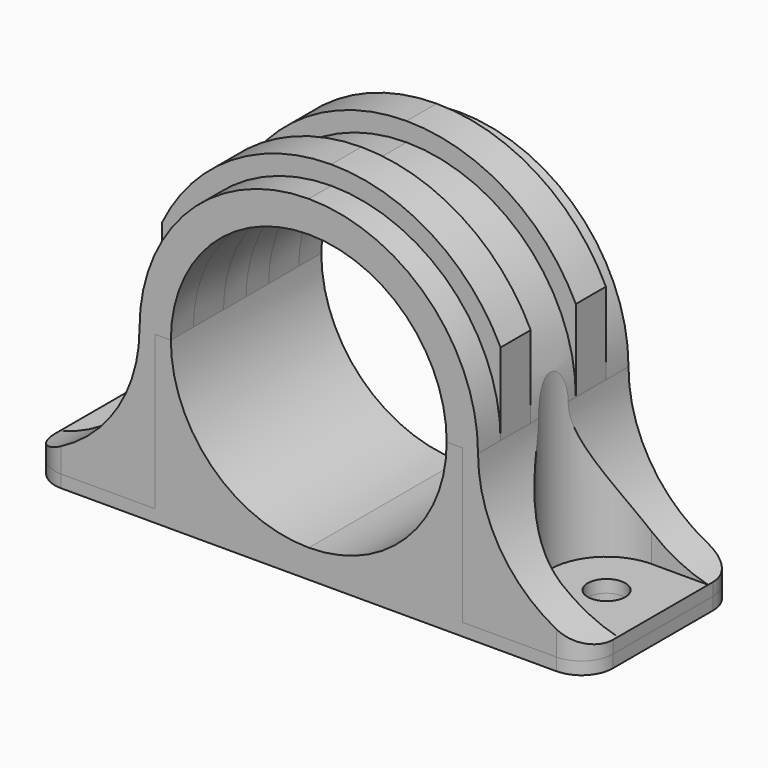
from build123d import *

# Parameters (mm, degrees)
F1_DEPTH       = 15
F1_DEPTH_BACK  = 15
F2_DEPTH       = 15
F2_DEPTH_BACK  = 15
F3_R           = 3
F4_DEPTH       = 53.501
F7_START       = -4
F6_R           = 3
F7_DEPTH       = 36
F9_W           = 6
F9_H           = 30
F10_DEPTH      = 27
F10_DEPTH_BACK = 27
F12_R          = 5
F12_2_R        = 5
F11_R          = 22
F13_DEPTH      = 25
F13_DEPTH_BACK = 25


with BuildPart() as f1:
    # F0 (on Front) → F1 (new body, two sides)
    with BuildSketch(Plane.XZ) as f1_sk:
        with BuildLine():
            Line((0, -26.5), (44.5, -26.5))
            Line((44.5, -26.5), (44.5, -24.5))
            Line((44.5, -24.5), (24.5, -24.5))
            Line((24.5, -24.5), (24.5, 0))
            Line((24.5, 0), (22, 0))
            ThreePointArc((22, 0), (15.5563491861, -15.5563491861), (0, -22))
            Line((0, -22), (0, -26.5))
        make_face()
    extrude(amount=F1_DEPTH)
    extrude(f1_sk.sketch, amount=-F1_DEPTH_BACK)


with BuildPart() as f2:
    # F0 (on Front) → F2 (new body, two sides)
    with BuildSketch(Plane.XZ) as f2_sk:
        with BuildLine():
            Line((24.5, -24.5), (44.5, -24.5))
            Line((44.5, -24.5), (44.5, -22.5))
            Line((44.5, -22.5), (27, -22.5))
            Line((27, -22.5), (27, 0))
            ThreePointArc((27, 0), (19.091883092, 19.091883092), (0, 27))
            Line((0, 27), (0, 22))
            ThreePointArc((0, 22), (15.5563491861, 15.5563491861), (22, 0))
            Line((22, 0), (24.5, 0))
            Line((24.5, 0), (24.5, -24.5))
        make_face()
        with BuildLine():
            Line((27, -22.5), (44.5, -22.5))
            ThreePointArc((44.5, -22.5), (31.8900378109, -14.2521928137), (27, 0))
            Line((27, 0), (27, -22.5))
        make_face()
    extrude(amount=F2_DEPTH)
    extrude(f2_sk.sketch, amount=-F2_DEPTH_BACK)


with BuildPart() as f4_tool:
    # F3 (on face) → F4 (new body, through all)
    with BuildSketch(Plane(origin=(0, 0, -26.5), x_dir=(1, 0, 0), z_dir=(0, 0, -1))):
        with Locations((35.4990586638, 0)):
            Circle(F3_R)
    extrude(amount=-F4_DEPTH)


with BuildPart() as f1_1:
    add(f1.part)

    # F4: cut by f4_tool
    add(f4_tool.part, mode=Mode.SUBTRACT)

    # F5: F1 across plane


with BuildPart() as f2_1:
    add(f2.part)

    # F4: cut by f4_tool
    add(f4_tool.part, mode=Mode.SUBTRACT)

    # F6 (on face) → F7 (cut)
    with BuildSketch(Plane(origin=(0, 0, -26.5), x_dir=(1, 0, 0), z_dir=(0, 0, -1)).offset(F7_START)):
        with BuildLine():
            Line((35.4990586638, -9), (44.5, -9))
            Line((44.5, -9), (44.4981174261, 9))
            Line((44.4981174261, 9), (35.4990586638, 9))
            ThreePointArc((35.4990586638, 9), (26.4990586638, 0), (35.4990586638, -9))
        make_face()
        with Locations((35.4990586638, 0)):
            Circle(F6_R, mode=Mode.SUBTRACT)
    extrude(amount=-F7_DEPTH, mode=Mode.SUBTRACT)

    # F8: F2 across plane


with BuildPart() as f1_2:
    add(f1_1.part)
    add(f1_1.part.mirror(Plane.YZ))

    # F12
    f12_edges = [f1_2.edges().sort_by_distance(p)[0] for p in [
        (-44.5, 15, -25.5),
        (-44.5, -15, -25.5),
        (44.5, -15, -25.5),
        (44.5, 15, -25.5),
    ]]
    fillet(f12_edges, radius=F12_R)


with BuildPart() as f2_2:
    add(f2_1.part)
    add(f2_1.part.mirror(Plane.YZ))

    # F9 (on Right) → F10 (join, two sides)
    with BuildSketch(Plane.YZ) as f10_sk:
        with Locations((7.5, 15)):
            Rectangle(F9_W, F9_H)
        with Locations((-7.5, 15)):
            Rectangle(F9_W, F9_H)
    extrude(amount=F10_DEPTH)
    extrude(f10_sk.sketch, amount=-F10_DEPTH_BACK)

    # F12#2
    f12_2_edges = [f2_2.edges().sort_by_distance(p)[0] for p in [
        (-44.5, 15, -23.5),
        (-44.5, -15, -23.5),
        (44.5, -15, -23.5),
        (44.5, 15, -23.5),
    ]]
    fillet(f12_2_edges, radius=F12_2_R)

    # F11 (on Front) → F13 (cut, two sides)
    with BuildSketch(Plane.XZ) as f13_sk:
        with BuildLine():
            Line((30, 0), (42, 0))
            ThreePointArc((42, 0), (0, 42), (-42, 0))
            Line((-42, 0), (-30, 0))
            ThreePointArc((-30, 0), (0, 30), (30, 0))
        make_face()
        Circle(F11_R)
    extrude(amount=-F13_DEPTH, mode=Mode.SUBTRACT)
    extrude(f13_sk.sketch, amount=F13_DEPTH_BACK, mode=Mode.SUBTRACT)


solid = Compound([f1_2.part, f2_2.part])
